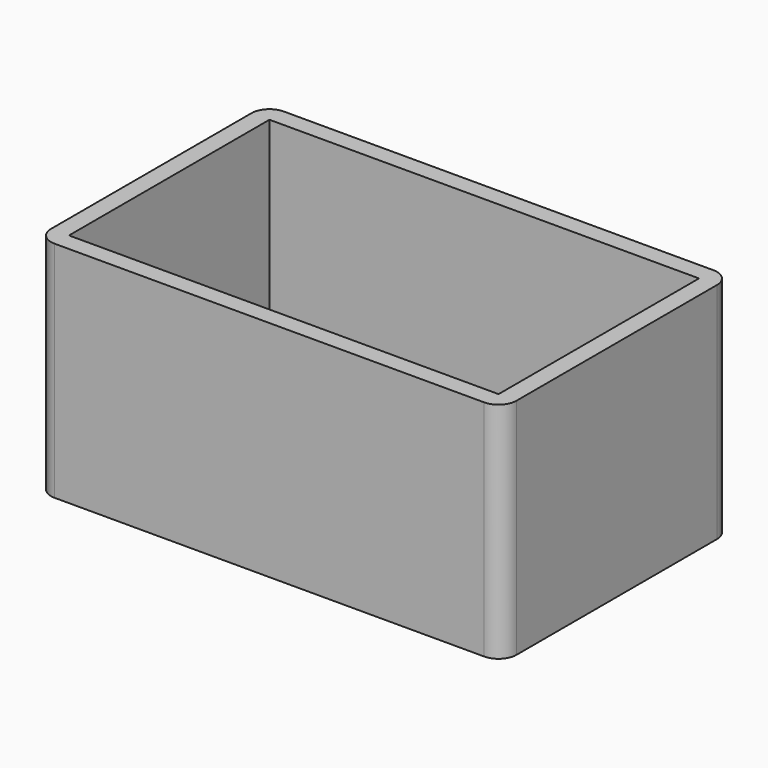
from build123d import *

# Parameters (mm, degrees)
F1_DEPTH = 25
F2_T     = 2
F4_W     = 10.5
F4_H     = 4
F5_DEPTH = 3


# Not quite as in the source:
# - a shell that OpenCascade refuses in one call is made with other operations: the cavity is built on its own and cut out


with BuildPart() as f1:
    # F0 (on Top) → F1 (new body)
    with BuildSketch(Plane.XY):
        with BuildLine():
            Line((24, 16), (-24, 16))
            ThreePointArc((-24, 16), (-25.4142135624, 15.4142135624), (-26, 14))
            Line((-26, 14), (-26, -14))
            ThreePointArc((-26, -14), (-25.4142135624, -15.4142135624), (-24, -16))
            Line((-24, -16), (24, -16))
            ThreePointArc((24, -16), (25.4142135624, -15.4142135624), (26, -14))
            Line((26, -14), (26, 14))
            ThreePointArc((26, 14), (25.4142135624, 15.4142135624), (24, 16))
        make_face()
    extrude(amount=F1_DEPTH)

    # F2: shell of thickness 2, made by hand


with BuildPart() as f2_core1:
    # F2_t2: copy of F1
    add(f1.part)

    # the walls: a layer under each face that stays
    f2_faces = [f2_core1.faces().sort_by_distance(p)[0] for p in [
        (0, 16, 12.5),
        (-26, 0, 12.5),
        (0, -16, 12.5),
        (26, 0, 12.5),
        (0, 0, 0),
    ]]
    thicken(f2_faces, amount=-F2_T, mode=Mode.SUBTRACT)


with BuildPart() as f1_1:
    add(f1.part)

    # what is left inside the walls is the cavity
    f2_cavity = [f2_core1.part.solids().sort_by_distance(p)[0] for p in [
        (0, -4.666667, 2.02),
    ]]
    add(f2_cavity, mode=Mode.SUBTRACT)

    # F4 (on offset) → F5 (cut)
    with BuildSketch(Plane.YZ.offset(25.5)):
        with Locations((0, 4)):
            Rectangle(F4_W, F4_H)
    extrude(amount=-F5_DEPTH, mode=Mode.SUBTRACT)


solid = f1_1.part
